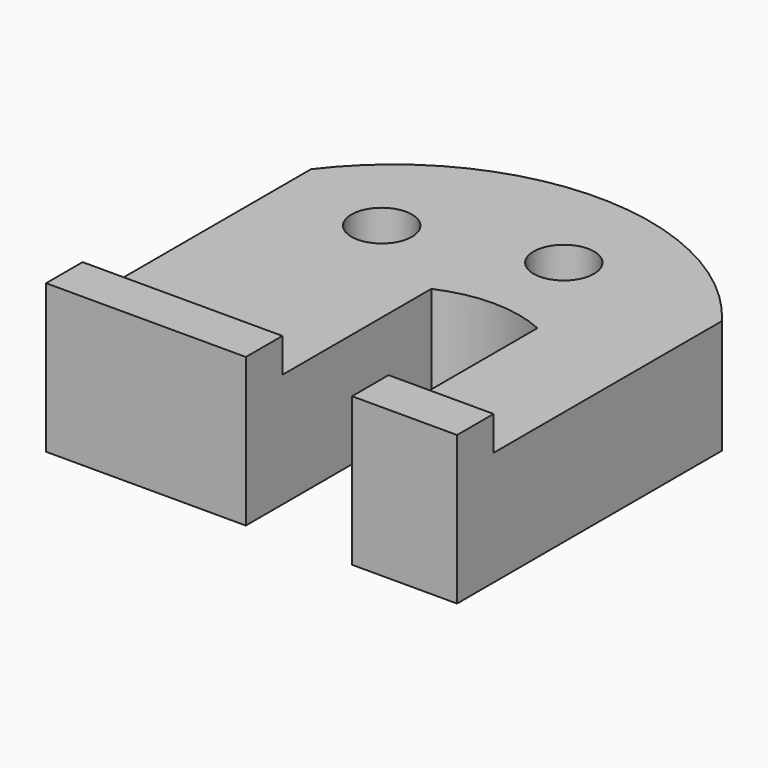
from build123d import *

# Parameters (mm, degrees)
F0_R     = 2.65
F1_DEPTH = 10
F2_W     = 9.2
F2_H     = 10
F2_H_2   = 3
F3_DEPTH = 4
F4_W     = 17.5
F4_H     = 10
F4_H_2   = 3
F5_DEPTH = 4


with BuildPart() as f1:
    # F0 (on Top) → F1 (new body)
    with BuildSketch(Plane.XY):
        with BuildLine():
            Line((-18, 7.8823786229), (-18, -17.1176213771))
            Line((-18, -17.1176213771), (-0.5, -17.1176213771))
            Line((-0.5, -17.1176213771), (-0.5, -0.8176213771))
            ThreePointArc((-0.5, -0.8176213771), (4.15, 0.1823786229), (8.8, -0.8176213771))
            Line((8.8, -0.8176213771), (8.8, -17.1176213771))
            Line((8.8, -17.1176213771), (18, -17.1176213771))
            Line((18, -17.1176213771), (18, 7.8823786229))
            ThreePointArc((18, 7.8823786229), (0, 16.8823786229), (-18, 7.8823786229))
        make_face()
        with Locations((-9, 4.3823786229)):
            Circle(F0_R, mode=Mode.SUBTRACT)
        with Locations((4.15, 7.8823786229)):
            Circle(F0_R, mode=Mode.SUBTRACT)
    extrude(amount=F1_DEPTH)

    # F2 (on face) → F3 (join)
    with BuildSketch(Plane.XZ.offset(17.1176213771)):
        with Locations((13.4, 5)):
            Rectangle(F2_W, F2_H)
        with Locations((13.4, 11.5)):
            Rectangle(F2_W, F2_H_2)
    extrude(amount=F3_DEPTH)

    # F4 (on face) → F5 (join, through all)
    with BuildSketch(Plane.XZ.offset(17.1176213771)):
        with Locations((-9.25, 5)):
            Rectangle(F4_W, F4_H)
        with Locations((-9.25, 11.5)):
            Rectangle(F4_W, F4_H_2)
    extrude(amount=F5_DEPTH)


solid = f1.part
